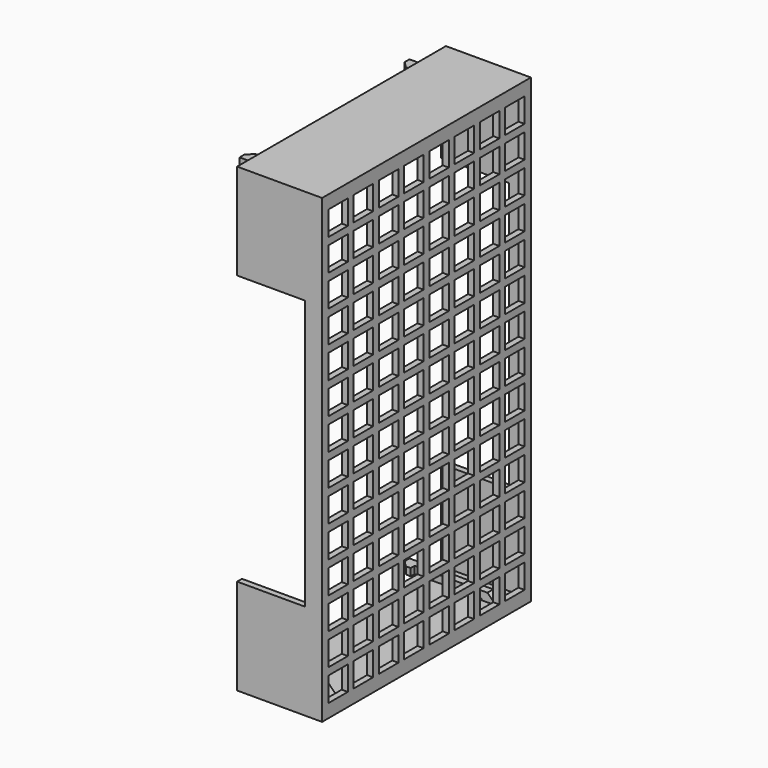
from build123d import *

# Parameters (mm, degrees)
F0_W      = 107.5
F0_H      = 190
F0_W_2    = 10
F0_H_2    = 10
F1_DEPTH  = 2.5
F2_W      = 107.5
F2_H      = 190
F2_W_2    = 102.5
F2_H_2    = 185
F3_DEPTH  = 32.5
F5_W      = 3
F5_H      = 3.5
F6_DEPTH  = 31
F7_SIZE2  = 3.49999
F7_SIZE   = 3.49999
F8_W      = 3
F8_H      = 0.5
F9_DEPTH  = 25
F10_DEPTH = 7
F11_W     = 4.5
F11_H     = 3
F12_DEPTH = 2
F13_SIZE2 = 2.5
F13_SIZE  = 2.5
F14_W     = 4.5
F14_H     = 3
F15_DEPTH = 2
F16_SIZE  = 2.5
F17_W     = 4.5
F17_H     = 3
F18_DEPTH = 2
F19_SIZE  = 2.5
F20_W     = 4.5
F20_H     = 3
F21_DEPTH = 2
F22_SIZE  = 2.5
F23_DEPTH = 107.5


# Not quite as in the source:
# - a fillet or chamfer is up to 0.001 mm smaller than in the source, because OpenCascade refuses the exact size


with BuildPart() as f1:
    # F0 (on Right) → F1 (new body)
    with BuildSketch(Plane.YZ):
        with Locations((-0.7359813899, 28.6250563264)):
            Rectangle(F0_W, F0_H)
        with Locations((-46.2359813899, -55.8749436736)):
            Rectangle(F0_W_2, F0_H_2, mode=Mode.SUBTRACT)
        with Locations((-46.2359813899, -42.8749436736)):
            Rectangle(F0_W_2, F0_H_2, mode=Mode.SUBTRACT)
        with Locations((-33.2359813899, -55.8749436736)):
            Rectangle(F0_W_2, F0_H_2, mode=Mode.SUBTRACT)
        with Locations((-33.2359813899, -42.8749436736)):
            Rectangle(F0_W_2, F0_H_2, mode=Mode.SUBTRACT)
        with Locations((-46.2359813899, -29.8749436736)):
            Rectangle(F0_W_2, F0_H_2, mode=Mode.SUBTRACT)
        with Locations((-33.2359813899, -29.8749436736)):
            Rectangle(F0_W_2, F0_H_2, mode=Mode.SUBTRACT)
        with Locations((-20.2359813899, -55.8749436736)):
            Rectangle(F0_W_2, F0_H_2, mode=Mode.SUBTRACT)
        with Locations((-20.2359813899, -42.8749436736)):
            Rectangle(F0_W_2, F0_H_2, mode=Mode.SUBTRACT)
        with Locations((-7.2359813899, -55.8749436736)):
            Rectangle(F0_W_2, F0_H_2, mode=Mode.SUBTRACT)
        with Locations((-7.2359813899, -42.8749436736)):
            Rectangle(F0_W_2, F0_H_2, mode=Mode.SUBTRACT)
        with Locations((-20.2359813899, -29.8749436736)):
            Rectangle(F0_W_2, F0_H_2, mode=Mode.SUBTRACT)
        with Locations((-7.2359813899, -29.8749436736)):
            Rectangle(F0_W_2, F0_H_2, mode=Mode.SUBTRACT)
        with Locations((-46.2359813899, -16.8749436736)):
            Rectangle(F0_W_2, F0_H_2, mode=Mode.SUBTRACT)
        with Locations((-46.2359813899, -3.8749436736)):
            Rectangle(F0_W_2, F0_H_2, mode=Mode.SUBTRACT)
        with Locations((-33.2359813899, -16.8749436736)):
            Rectangle(F0_W_2, F0_H_2, mode=Mode.SUBTRACT)
        with Locations((-33.2359813899, -3.8749436736)):
            Rectangle(F0_W_2, F0_H_2, mode=Mode.SUBTRACT)
        with Locations((-46.2359813899, 9.1250563264)):
            Rectangle(F0_W_2, F0_H_2, mode=Mode.SUBTRACT)
        with Locations((-46.2359813899, 22.1250563264)):
            Rectangle(F0_W_2, F0_H_2, mode=Mode.SUBTRACT)
        with Locations((-33.2359813899, 9.1250563264)):
            Rectangle(F0_W_2, F0_H_2, mode=Mode.SUBTRACT)
        with Locations((-33.2359813899, 22.1250563264)):
            Rectangle(F0_W_2, F0_H_2, mode=Mode.SUBTRACT)
        with Locations((-20.2359813899, -16.8749436736)):
            Rectangle(F0_W_2, F0_H_2, mode=Mode.SUBTRACT)
        with Locations((-20.2359813899, -3.8749436736)):
            Rectangle(F0_W_2, F0_H_2, mode=Mode.SUBTRACT)
        with Locations((-7.2359813899, -16.8749436736)):
            Rectangle(F0_W_2, F0_H_2, mode=Mode.SUBTRACT)
        with Locations((-7.2359813899, -3.8749436736)):
            Rectangle(F0_W_2, F0_H_2, mode=Mode.SUBTRACT)
        with Locations((-20.2359813899, 9.1250563264)):
            Rectangle(F0_W_2, F0_H_2, mode=Mode.SUBTRACT)
        with Locations((-20.2359813899, 22.1250563264)):
            Rectangle(F0_W_2, F0_H_2, mode=Mode.SUBTRACT)
        with Locations((-7.2359813899, 9.1250563264)):
            Rectangle(F0_W_2, F0_H_2, mode=Mode.SUBTRACT)
        with Locations((-7.2359813899, 22.1250563264)):
            Rectangle(F0_W_2, F0_H_2, mode=Mode.SUBTRACT)
        with Locations((5.7640186101, -55.8749436736)):
            Rectangle(F0_W_2, F0_H_2, mode=Mode.SUBTRACT)
        with Locations((5.7640186101, -42.8749436736)):
            Rectangle(F0_W_2, F0_H_2, mode=Mode.SUBTRACT)
        with Locations((18.7640186101, -55.8749436736)):
            Rectangle(F0_W_2, F0_H_2, mode=Mode.SUBTRACT)
        with Locations((18.7640186101, -42.8749436736)):
            Rectangle(F0_W_2, F0_H_2, mode=Mode.SUBTRACT)
        with Locations((5.7640186101, -29.8749436736)):
            Rectangle(F0_W_2, F0_H_2, mode=Mode.SUBTRACT)
        with Locations((18.7640186101, -29.8749436736)):
            Rectangle(F0_W_2, F0_H_2, mode=Mode.SUBTRACT)
        with Locations((31.7640186101, -55.8749436736)):
            Rectangle(F0_W_2, F0_H_2, mode=Mode.SUBTRACT)
        with Locations((31.7640186101, -42.8749436736)):
            Rectangle(F0_W_2, F0_H_2, mode=Mode.SUBTRACT)
        with Locations((44.7640186101, -55.8749436736)):
            Rectangle(F0_W_2, F0_H_2, mode=Mode.SUBTRACT)
        with Locations((44.7640186101, -42.8749436736)):
            Rectangle(F0_W_2, F0_H_2, mode=Mode.SUBTRACT)
        with Locations((31.7640186101, -29.8749436736)):
            Rectangle(F0_W_2, F0_H_2, mode=Mode.SUBTRACT)
        with Locations((44.7640186101, -29.8749436736)):
            Rectangle(F0_W_2, F0_H_2, mode=Mode.SUBTRACT)
        with Locations((5.7640186101, -16.8749436736)):
            Rectangle(F0_W_2, F0_H_2, mode=Mode.SUBTRACT)
        with Locations((5.7640186101, -3.8749436736)):
            Rectangle(F0_W_2, F0_H_2, mode=Mode.SUBTRACT)
        with Locations((18.7640186101, -16.8749436736)):
            Rectangle(F0_W_2, F0_H_2, mode=Mode.SUBTRACT)
        with Locations((18.7640186101, -3.8749436736)):
            Rectangle(F0_W_2, F0_H_2, mode=Mode.SUBTRACT)
        with Locations((5.7640186101, 9.1250563264)):
            Rectangle(F0_W_2, F0_H_2, mode=Mode.SUBTRACT)
        with Locations((5.7640186101, 22.1250563264)):
            Rectangle(F0_W_2, F0_H_2, mode=Mode.SUBTRACT)
        with Locations((18.7640186101, 9.1250563264)):
            Rectangle(F0_W_2, F0_H_2, mode=Mode.SUBTRACT)
        with Locations((18.7640186101, 22.1250563264)):
            Rectangle(F0_W_2, F0_H_2, mode=Mode.SUBTRACT)
        with Locations((31.7640186101, -16.8749436736)):
            Rectangle(F0_W_2, F0_H_2, mode=Mode.SUBTRACT)
        with Locations((31.7640186101, -3.8749436736)):
            Rectangle(F0_W_2, F0_H_2, mode=Mode.SUBTRACT)
        with Locations((44.7640186101, -16.8749436736)):
            Rectangle(F0_W_2, F0_H_2, mode=Mode.SUBTRACT)
        with Locations((44.7640186101, -3.8749436736)):
            Rectangle(F0_W_2, F0_H_2, mode=Mode.SUBTRACT)
        with Locations((31.7640186101, 9.1250563264)):
            Rectangle(F0_W_2, F0_H_2, mode=Mode.SUBTRACT)
        with Locations((31.7640186101, 22.1250563264)):
            Rectangle(F0_W_2, F0_H_2, mode=Mode.SUBTRACT)
        with Locations((44.7640186101, 9.1250563264)):
            Rectangle(F0_W_2, F0_H_2, mode=Mode.SUBTRACT)
        with Locations((44.7640186101, 22.1250563264)):
            Rectangle(F0_W_2, F0_H_2, mode=Mode.SUBTRACT)
        with Locations((-46.2359813899, 35.1250563264)):
            Rectangle(F0_W_2, F0_H_2, mode=Mode.SUBTRACT)
        with Locations((-46.2359813899, 48.1250563264)):
            Rectangle(F0_W_2, F0_H_2, mode=Mode.SUBTRACT)
        with Locations((-33.2359813899, 35.1250563264)):
            Rectangle(F0_W_2, F0_H_2, mode=Mode.SUBTRACT)
        with Locations((-33.2359813899, 48.1250563264)):
            Rectangle(F0_W_2, F0_H_2, mode=Mode.SUBTRACT)
        with Locations((-46.2359813899, 61.1250563264)):
            Rectangle(F0_W_2, F0_H_2, mode=Mode.SUBTRACT)
        with Locations((-46.2359813899, 74.1250563264)):
            Rectangle(F0_W_2, F0_H_2, mode=Mode.SUBTRACT)
        with Locations((-33.2359813899, 61.1250563264)):
            Rectangle(F0_W_2, F0_H_2, mode=Mode.SUBTRACT)
        with Locations((-33.2359813899, 74.1250563264)):
            Rectangle(F0_W_2, F0_H_2, mode=Mode.SUBTRACT)
        with Locations((-20.2359813899, 35.1250563264)):
            Rectangle(F0_W_2, F0_H_2, mode=Mode.SUBTRACT)
        with Locations((-20.2359813899, 48.1250563264)):
            Rectangle(F0_W_2, F0_H_2, mode=Mode.SUBTRACT)
        with Locations((-7.2359813899, 35.1250563264)):
            Rectangle(F0_W_2, F0_H_2, mode=Mode.SUBTRACT)
        with Locations((-7.2359813899, 48.1250563264)):
            Rectangle(F0_W_2, F0_H_2, mode=Mode.SUBTRACT)
        with Locations((-20.2359813899, 61.1250563264)):
            Rectangle(F0_W_2, F0_H_2, mode=Mode.SUBTRACT)
        with Locations((-20.2359813899, 74.1250563264)):
            Rectangle(F0_W_2, F0_H_2, mode=Mode.SUBTRACT)
        with Locations((-7.2359813899, 61.1250563264)):
            Rectangle(F0_W_2, F0_H_2, mode=Mode.SUBTRACT)
        with Locations((-7.2359813899, 74.1250563264)):
            Rectangle(F0_W_2, F0_H_2, mode=Mode.SUBTRACT)
        with Locations((-46.2359813899, 87.1250563264)):
            Rectangle(F0_W_2, F0_H_2, mode=Mode.SUBTRACT)
        with Locations((-33.2359813899, 87.1250563264)):
            Rectangle(F0_W_2, F0_H_2, mode=Mode.SUBTRACT)
        with Locations((-46.2359813899, 100.1250563264)):
            Rectangle(F0_W_2, F0_H_2, mode=Mode.SUBTRACT)
        with Locations((-46.2359813899, 113.1250563264)):
            Rectangle(F0_W_2, F0_H_2, mode=Mode.SUBTRACT)
        with Locations((-33.2359813899, 100.1250563264)):
            Rectangle(F0_W_2, F0_H_2, mode=Mode.SUBTRACT)
        with Locations((-33.2359813899, 113.1250563264)):
            Rectangle(F0_W_2, F0_H_2, mode=Mode.SUBTRACT)
        with Locations((-20.2359813899, 87.1250563264)):
            Rectangle(F0_W_2, F0_H_2, mode=Mode.SUBTRACT)
        with Locations((-7.2359813899, 87.1250563264)):
            Rectangle(F0_W_2, F0_H_2, mode=Mode.SUBTRACT)
        with Locations((-20.2359813899, 100.1250563264)):
            Rectangle(F0_W_2, F0_H_2, mode=Mode.SUBTRACT)
        with Locations((-20.2359813899, 113.1250563264)):
            Rectangle(F0_W_2, F0_H_2, mode=Mode.SUBTRACT)
        with Locations((-7.2359813899, 100.1250563264)):
            Rectangle(F0_W_2, F0_H_2, mode=Mode.SUBTRACT)
        with Locations((-7.2359813899, 113.1250563264)):
            Rectangle(F0_W_2, F0_H_2, mode=Mode.SUBTRACT)
        with Locations((5.7640186101, 35.1250563264)):
            Rectangle(F0_W_2, F0_H_2, mode=Mode.SUBTRACT)
        with Locations((5.7640186101, 48.1250563264)):
            Rectangle(F0_W_2, F0_H_2, mode=Mode.SUBTRACT)
        with Locations((18.7640186101, 35.1250563264)):
            Rectangle(F0_W_2, F0_H_2, mode=Mode.SUBTRACT)
        with Locations((18.7640186101, 48.1250563264)):
            Rectangle(F0_W_2, F0_H_2, mode=Mode.SUBTRACT)
        with Locations((5.7640186101, 61.1250563264)):
            Rectangle(F0_W_2, F0_H_2, mode=Mode.SUBTRACT)
        with Locations((5.7640186101, 74.1250563264)):
            Rectangle(F0_W_2, F0_H_2, mode=Mode.SUBTRACT)
        with Locations((18.7640186101, 61.1250563264)):
            Rectangle(F0_W_2, F0_H_2, mode=Mode.SUBTRACT)
        with Locations((18.7640186101, 74.1250563264)):
            Rectangle(F0_W_2, F0_H_2, mode=Mode.SUBTRACT)
        with Locations((31.7640186101, 35.1250563264)):
            Rectangle(F0_W_2, F0_H_2, mode=Mode.SUBTRACT)
        with Locations((31.7640186101, 48.1250563264)):
            Rectangle(F0_W_2, F0_H_2, mode=Mode.SUBTRACT)
        with Locations((44.7640186101, 35.1250563264)):
            Rectangle(F0_W_2, F0_H_2, mode=Mode.SUBTRACT)
        with Locations((44.7640186101, 48.1250563264)):
            Rectangle(F0_W_2, F0_H_2, mode=Mode.SUBTRACT)
        with Locations((31.7640186101, 61.1250563264)):
            Rectangle(F0_W_2, F0_H_2, mode=Mode.SUBTRACT)
        with Locations((31.7640186101, 74.1250563264)):
            Rectangle(F0_W_2, F0_H_2, mode=Mode.SUBTRACT)
        with Locations((44.7640186101, 61.1250563264)):
            Rectangle(F0_W_2, F0_H_2, mode=Mode.SUBTRACT)
        with Locations((44.7640186101, 74.1250563264)):
            Rectangle(F0_W_2, F0_H_2, mode=Mode.SUBTRACT)
        with Locations((5.7640186101, 87.1250563264)):
            Rectangle(F0_W_2, F0_H_2, mode=Mode.SUBTRACT)
        with Locations((18.7640186101, 87.1250563264)):
            Rectangle(F0_W_2, F0_H_2, mode=Mode.SUBTRACT)
        with Locations((5.7640186101, 100.1250563264)):
            Rectangle(F0_W_2, F0_H_2, mode=Mode.SUBTRACT)
        with Locations((5.7640186101, 113.1250563264)):
            Rectangle(F0_W_2, F0_H_2, mode=Mode.SUBTRACT)
        with Locations((18.7640186101, 100.1250563264)):
            Rectangle(F0_W_2, F0_H_2, mode=Mode.SUBTRACT)
        with Locations((18.7640186101, 113.1250563264)):
            Rectangle(F0_W_2, F0_H_2, mode=Mode.SUBTRACT)
        with Locations((31.7640186101, 87.1250563264)):
            Rectangle(F0_W_2, F0_H_2, mode=Mode.SUBTRACT)
        with Locations((44.7640186101, 87.1250563264)):
            Rectangle(F0_W_2, F0_H_2, mode=Mode.SUBTRACT)
        with Locations((31.7640186101, 100.1250563264)):
            Rectangle(F0_W_2, F0_H_2, mode=Mode.SUBTRACT)
        with Locations((31.7640186101, 113.1250563264)):
            Rectangle(F0_W_2, F0_H_2, mode=Mode.SUBTRACT)
        with Locations((44.7640186101, 100.1250563264)):
            Rectangle(F0_W_2, F0_H_2, mode=Mode.SUBTRACT)
        with Locations((44.7640186101, 113.1250563264)):
            Rectangle(F0_W_2, F0_H_2, mode=Mode.SUBTRACT)
    extrude(amount=F1_DEPTH)

    # F2 (on face) → F3 (join)
    with BuildSketch(Plane(origin=(0, 0, 0), x_dir=(0, -1, 0), z_dir=(-1, 0, 0))):
        with Locations((0.7359813899, 28.6250563264)):
            Rectangle(F2_W, F2_H)
        with Locations((0.7359813899, 28.6250563264)):
            Rectangle(F2_W_2, F2_H_2, mode=Mode.SUBTRACT)
    extrude(amount=F3_DEPTH)

    # F5 (on face) → F6 (join)
    with BuildSketch(Plane(origin=(-32.5, 0, 0), x_dir=(0, -1, 0), z_dir=(-1, 0, 0))):
        with Locations((-41.5140186101, 119.3750563264)):
            Rectangle(F5_W, F5_H)
        with Locations((42.9859813899, 119.3750563264)):
            Rectangle(F5_W, F5_H)
        with Locations((-41.5140186101, -62.1249436736)):
            Rectangle(F5_W, F5_H)
        with Locations((42.9859813899, -62.1249436736)):
            Rectangle(F5_W, F5_H)
    extrude(amount=-F6_DEPTH)

    # F7 (size 3.5 and 3.5 in the source; OpenCascade refuses exactly that, so slightly less here)
    f7_edges = [f1.edges().sort_by_distance(p)[0] for p in [
        (-1.5, -42.985981, -60.374944),
        (-1.5, 41.514019, -60.374944),
        (-1.5, 41.514019, 117.625056),
        (-1.5, -42.985981, 117.625056),
    ]]
    chamfer(f7_edges, length=F7_SIZE, length2=F7_SIZE2)

    # F8 (on face) → F9 (cut)
    with BuildSketch(Plane(origin=(-32.5, 0, 0), x_dir=(0, -1, 0), z_dir=(-1, 0, 0))):
        with Locations((-41.5140186101, -63.6249436736)):
            Rectangle(F8_W, F8_H)
        with Locations((42.9859813899, -63.6249436736)):
            Rectangle(F8_W, F8_H)
        with Locations((-41.5140186101, 120.8750563264)):
            Rectangle(F8_W, F8_H)
        with Locations((42.9859813899, 120.8750563264)):
            Rectangle(F8_W, F8_H)
    extrude(amount=-F9_DEPTH, mode=Mode.SUBTRACT)

    # F10 (add): faces of the model
    f10_faces = [f1.faces().sort_by_distance(p)[0] for p in [
        (-32.5, 41.5140186101, 119.1250563264),
        (-32.5, -42.9859813899, 119.1250563264),
        (-32.5, 41.5140186101, -61.8749436736),
        (-32.5, -42.9859813899, -61.8749436736),
    ]]
    extrude(f10_faces, amount=F10_DEPTH)

    # F11 (on face) → F12 (join)
    with BuildSketch(Plane.XZ.offset(-40.0140186101)):
        with Locations((-37.25, 119.1250563264)):
            Rectangle(F11_W, F11_H)
    extrude(amount=F12_DEPTH)

    # F13
    f13_edges = [f1.edges().sort_by_distance(p)[0] for p in [
        (-39.5, 38.014019, 119.125056),
    ]]
    chamfer(f13_edges, length=F13_SIZE, length2=F13_SIZE2)

    # F14 (on face) → F15 (join)
    with BuildSketch(Plane.XZ.offset(-40.0140186101)):
        with Locations((-37.25, -61.8749436736)):
            Rectangle(F14_W, F14_H)
    extrude(amount=F15_DEPTH)

    # F16
    f16_edges = [f1.edges().sort_by_distance(p)[0] for p in [
        (-39.5, 38.014019, -61.874944),
    ]]
    chamfer(f16_edges, length=F16_SIZE)

    # F17 (on face) → F18 (join)
    with BuildSketch(Plane(origin=(0, -41.4859813899, 0), x_dir=(-1, 0, 0), z_dir=(0, 1, 0))):
        with Locations((37.25, 119.1250563264)):
            Rectangle(F17_W, F17_H)
    extrude(amount=F18_DEPTH)

    # F19
    f19_edges = [f1.edges().sort_by_distance(p)[0] for p in [
        (-39.5, -39.485981, 119.125056),
    ]]
    chamfer(f19_edges, length=F19_SIZE)

    # F20 (on face) → F21 (join)
    with BuildSketch(Plane(origin=(0, -41.4859813899, 0), x_dir=(-1, 0, 0), z_dir=(0, 1, 0))):
        with Locations((37.25, -61.8749436736)):
            Rectangle(F20_W, F20_H)
    extrude(amount=F21_DEPTH)

    # F22
    f22_edges = [f1.edges().sort_by_distance(p)[0] for p in [
        (-39.5, -39.485981, -61.874944),
    ]]
    chamfer(f22_edges, length=F22_SIZE)

    # F4 (on face) → F23 (cut)
    with BuildSketch(Plane.XZ.offset(54.4859813899)):
        Polygon((-4.5, -26.8749436736), (-4.5, 28.6250563264), (-4.5, 84.1250563264), (-32.5, 84.1250563264), (-32.5, 28.6250563264), (-32.5, -26.8749436736), align=None)
    extrude(amount=-F23_DEPTH, mode=Mode.SUBTRACT)


solid = f1.part
